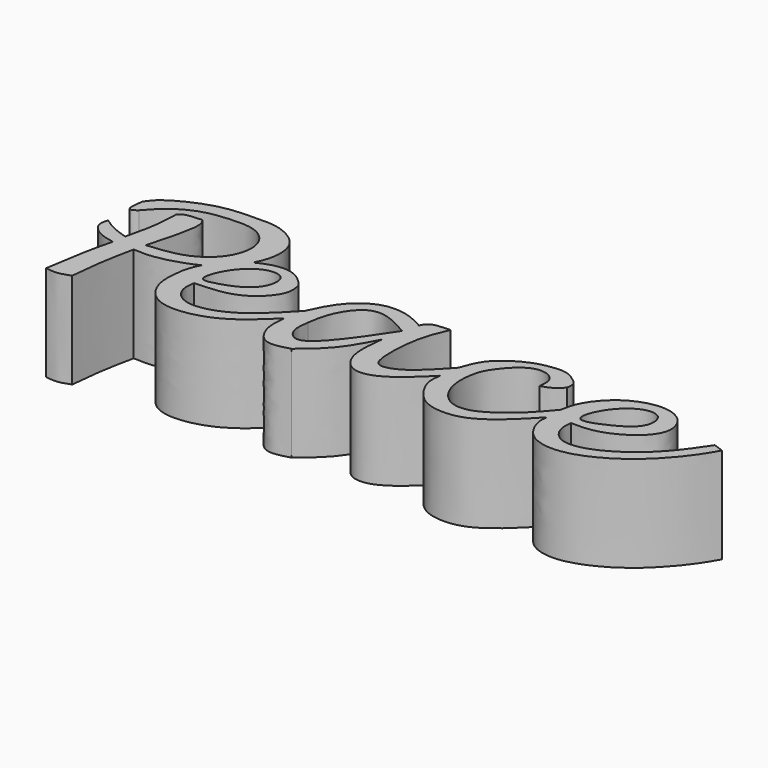
from build123d import *

# Parameters (mm, degrees)
F1_DEPTH = 15


with BuildPart() as f1:
    # F0 (on Top) → F1 (new body)
    with BuildSketch(Plane.XY):
        with BuildLine():
            add(Edge.make_bspline(
                [(-29.5197498053, 16.0896964371), (-29.2959248841, 17.0866768453), (-28.9570431175, 17.9865364975), (-28.5339232006, 18.7932092998)],
                knots=[0, 0, 0, 0, 0.1193114698, 0.1193114698, 0.1193114698, 0.1193114698], degree=3))
            add(Edge.make_bspline(
                [(-29.5197498053, 16.0896964371), (-29.7031065197, 14.6563172426), (-30.080045439, 11.7096217462), (-28.1322871252, 8.759925381), (-26.4865215868, 8.0765383318)],
                knots=[0, 0, 0, 0, 0.2073575456, 0.4262790671, 0.4262790671, 0.4262790671, 0.4262790671], degree=3))
            add(Edge.make_bspline(
                [(-26.4865215868, 8.0765383318), (-24.3712413413, 7.1981901762), (-17.8840994319, 8.2079095342), (-13.895871726, 12.139582434), (-11.8636386469, 14.1429975629)],
                knots=[0.4262790671, 0.4262790671, 0.4262790671, 0.4262790671, 0.7076559455, 1, 1, 1, 1], degree=3))
            add(Edge.make_bspline(
                [(-11.8636386469, 14.1429975629), (-11.9919670944, 13.0883304188), (-12.2526083771, 10.9462504463), (-10.2153785321, 7.2023382975), (-7.5198727613, 7.9751970563), (-6.1371922493, 8.3716409281)],
                knots=[0, 0, 0, 0, 0.3208255575, 0.6516122221, 1, 1, 1, 1], degree=3))
            add(Edge.make_bspline(
                [(-6.1371922493, 8.3716409281), (-4.7049770612, 9.5508191577), (-1.8004106416, 11.944123887), (0.0085061179, 15.4262155687), (0.9252529708, 17.1948950738)],
                knots=[0, 0, 0, 0, 0.4928718937, 1, 1, 1, 1], degree=3))
            add(Edge.make_bspline(
                [(0.9252529708, 17.1948950738), (0.7002885074, 15.2129187205), (0.2948956357, 11.6686773245), (2.8534995196, 8.3256503296), (7.2214848398, 9.0430540833), (10.5903189017, 12.2451424426), (12.4796722084, 14.1429975629)],
                knots=[0, 0, 0, 0, 0.2662560325, 0.4748550688, 0.6918347611, 1, 1, 1, 1], degree=3))
            add(Edge.make_bspline(
                [(12.4796722084, 14.1429975629), (12.3567270292, 13.3382773369), (12.14040693, 11.6866274324), (14.1680771363, 8.3563764669), (16.6960843798, 6.843858018), (20.9356335968, 6.7199377707), (25.0508891214, 9.0723771082), (28.001238583, 12.0543664551), (29.5260921121, 13.7017956004)],
                knots=[0, 0, 0, 0, 0.1309459503, 0.2919621729, 0.4354540719, 0.6027228467, 0.784505056, 1, 1, 1, 1], degree=3))
            add(Edge.make_bspline(
                [(29.5260921121, 13.7017956004), (29.4494344459, 13.1510419203), (29.3115775332, 11.9578711835), (31.001212058, 8.2394328011), (36.1145843581, 7.0708416903), (42.2117822652, 9.6169760573), (46.573863691, 13.1346350854), (49.9266045093, 17.0857546913), (51.1581874034, 19.2222665215), (51.7203956842, 20.1976578683)],
                knots=[0, 0, 0, 0, 0.0899502167, 0.2212376244, 0.3723173697, 0.5483148575, 0.7139379788, 0.8700324828, 1, 1, 1, 1], degree=3))
            Line((51.7203956842, 20.1976578683), (50.1595586538, 20.7686945796))
            add(Edge.make_bspline(
                [(32.7983126044, 14.3592404202), (32.7153503568, 13.7323555449), (32.5362242327, 12.3788307643), (34.177987249, 9.747083146), (38.8427355373, 9.7604999377), (45.8804799663, 14.4091846262), (48.7479970496, 18.6708504577), (50.1595586538, 20.7686945796)],
                knots=[0, 0, 0, 0, 0.130090907, 0.2808829393, 0.4700062965, 0.7391057348, 1, 1, 1, 1], degree=3))
            add(Edge.make_bspline(
                [(29.588283971, 16.3035858423), (29.7616917917, 17.2053776187), (30.1627716399, 19.291157298), (33.5068853144, 23.2810073199), (38.1596043126, 24.8599408195), (41.2541002931, 24.2873570254), (43.0490114044, 22.683768941), (43.7218716906, 20.0178969278), (41.6710895913, 16.88834866), (36.7785570041, 14.2784160551), (34.0517720177, 14.3337871939), (32.7983126044, 14.3592404202)],
                knots=[0, 0, 0, 0, 0.1000330229, 0.231369205, 0.3598860143, 0.4603773571, 0.5477091259, 0.6387126974, 0.7479317597, 0.8841282645, 1, 1, 1, 1], degree=3))
            add(Edge.make_bspline(
                [(23.645831272, 19.6124818176), (23.7203833838, 20.2123241708), (23.8704148875, 21.3933142156), (22.6701217375, 22.8924812944), (19.5221839217, 23.1427632594), (16.3109184961, 19.4772592399), (15.2895614031, 17.2986171252), (14.8792866219, 13.0982142101), (17.05717861, 9.3483199148), (21.2088747712, 8.5887501402), (26.7442270709, 12.8463793621), (28.7028105399, 15.2281055095), (29.588283971, 16.3035858423)],
                knots=[0, 0, 0, 0, 0.0707743039, 0.1396140029, 0.228929762, 0.3440556474, 0.4292761333, 0.536753367, 0.6438866817, 0.7459339665, 0.8852224949, 1, 1, 1, 1], degree=3))
            add(Edge.make_bspline(
                [(26.526927948, 21.3411394507), (26.1385483593, 20.9400395262), (25.3505362754, 20.126218212), (24.2194502874, 19.7853498294), (23.645831272, 19.6124818176)],
                knots=[0, 0, 0, 0, 0.4928599404, 1, 1, 1, 1], degree=3))
            add(Edge.make_bspline(
                [(12.8943044692, 17.1948950738), (13.3425896626, 18.491787842), (14.2804655004, 21.2142228005), (18.8593458781, 23.903692294), (21.393850445, 24.4249510687), (24.0737893185, 24.6930231444), (25.7581339132, 23.4584551751), (26.7110830768, 22.704102983), (26.5899543358, 21.8076092017), (26.526927948, 21.3411394507)],
                knots=[0, 0, 0, 0, 0.1840283222, 0.3856193225, 0.5329945244, 0.6763715981, 0.8040129767, 0.8980060108, 1, 1, 1, 1], degree=3))
            add(Edge.make_bspline(
                [(5.9051825665, 24.39795807), (5.2796526411, 22.9712299099), (3.9353644531, 19.9050894014), (3.7075616843, 12.9009672388), (4.9490431647, 11.3184163953), (8.496299722, 12.3856851943), (11.2468870531, 15.3909715866), (12.8943044692, 17.1948950738)],
                knots=[0, 0, 0, 0, 0.2170119072, 0.4664184993, 0.5823552154, 0.7497429619, 1, 1, 1, 1], degree=3))
            add(Edge.make_bspline(
                [(2.1475991234, 22.9039788246), (2.3428401586, 23.3003573055), (2.8310561944, 24.2915338294), (4.7522735677, 24.358045116), (5.9051825665, 24.39795807)],
                knots=[0, 0, 0, 0, 0.3999070512, 1, 1, 1, 1], degree=3))
            add(Edge.make_bspline(
                [(-11.1623937264, 17.1948950738), (-10.5398511892, 18.5628349484), (-9.2707374001, 21.3594980591), (-5.248213519, 24.7374533554), (-0.7298831893, 24.4906309653), (1.2322453903, 23.4086829672), (2.1475991234, 22.9039788246)],
                knots=[0, 0, 0, 0, 0.2603156398, 0.5312425545, 0.7812722516, 1, 1, 1, 1], degree=3))
            add(Edge.make_bspline(
                [(-26.3120550662, 14.4988177344), (-26.4222931202, 13.7768911895), (-26.6615542892, 12.2101495597), (-24.3282508745, 9.2469865739), (-17.4297661724, 10.5963680293), (-13.3925098593, 14.8444387075), (-11.1623937264, 17.1948950738)],
                knots=[0, 0, 0, 0, 0.1694155161, 0.367717612, 0.6506295652, 1, 1, 1, 1], degree=3))
            add(Edge.make_bspline(
                [(-15.95112037, 21.9937769871), (-15.7966520892, 21.216655299), (-15.4154688091, 19.2989425314), (-19.5008131736, 14.743263195), (-23.9492657643, 14.5836147697), (-26.3120550662, 14.4988177344)],
                knots=[0, 0, 0, 0, 0.2421048194, 0.5974450468, 1, 1, 1, 1], degree=3))
            add(Edge.make_bspline(
                [(-24.0700956622, 23.2628666258), (-23.2776920759, 23.6864516212), (-20.1311153039, 24.8738854789), (-17.7451969535, 24.2725213112), (-15.95112037, 21.9937769871)],
                knots=[0.4293270672, 0.4293270672, 0.4293270672, 0.4293270672, 0.5741513965, 1, 1, 1, 1], degree=3))
            add(Edge.make_bspline(
                [(-28.5339232006, 18.7932092998), (-27.4805344869, 19.3586454328), (-25.8445145474, 20.5733086864), (-24.5247192992, 22.4099469585), (-24.0700956622, 23.2628666258)],
                knots=[0.2164607486, 0.2164607486, 0.2164607486, 0.2164607486, 0.2921979477, 0.349944774, 0.349944774, 0.349944774, 0.349944774], degree=3))
        make_face()
        with BuildLine():
            add(Edge.make_bspline(
                [(-26.1831432581, 16.0770304501), (-26.5705475824, 16.5915824541), (-25.5236781222, 19.8500439887), (-22.3942558617, 22.7980811841), (-19.5909944076, 22.9806135847), (-18.455931748, 21.7897345319), (-18.7610605958, 19.3004890899), (-20.8794412927, 17.1979951748), (-24.0654910281, 16.0934411171), (-25.8961329296, 15.6958221609), (-26.1831432581, 16.0770304501)],
                knots=[0, 0, 0, 0, 0.1402941833, 0.3022737646, 0.4209424648, 0.5087922195, 0.6222593339, 0.7517086902, 0.8960623898, 1, 1, 1, 1], degree=3))
        make_face(mode=Mode.SUBTRACT)
        with BuildLine():
            add(Edge.make_bspline(
                [(-8.9235752821, 15.0464298204), (-9.0646859983, 14.0808295866), (-9.3271993781, 12.2844884749), (-7.5404688212, 10.3547407663), (-5.0207003169, 11.4635558948), (-1.2953094882, 16.3396092098), (0.5618805634, 19.1479797333), (1.4483764535, 20.4885043204)],
                knots=[0, 0, 0, 0, 0.1779548177, 0.3310557971, 0.4918670148, 0.7574519621, 1, 1, 1, 1], degree=3))
            add(Edge.make_bspline(
                [(-8.9235752821, 15.0464298204), (-8.7718449134, 16.1215699221), (-8.449567237, 18.4051843159), (-5.958882275, 22.3564152791), (-2.6113827935, 22.7845317726), (-0.0046509708, 21.3102749358), (1.4483764535, 20.4885043204)],
                knots=[0, 0, 0, 0, 0.2372477596, 0.5039179524, 0.7234771856, 1, 1, 1, 1], degree=3))
        make_face(mode=Mode.SUBTRACT)
        with BuildLine():
            add(Edge.make_bspline(
                [(32.9581163824, 15.9508809447), (32.4202349789, 16.4558861758), (33.5372547907, 19.9580854994), (37.2715590249, 23.1501136882), (40.5087156051, 22.7034723084), (40.7973008496, 19.1294802461), (37.0761086127, 16.8016116704), (33.520287852, 15.4230702953), (32.9581163824, 15.9508809447)],
                knots=[0, 0, 0, 0, 0.1648006178, 0.3622570844, 0.4996763079, 0.6407463677, 0.8277571879, 1, 1, 1, 1], degree=3))
        make_face(mode=Mode.SUBTRACT)
        with BuildLine():
            add(Edge.make_bspline(
                [(-37.63435781, 16.8396867812), (-36.792774095, 16.780997693), (-34.7988064496, 16.6419460296), (-30.9505530887, 17.6314034567), (-28.9442923194, 18.5729320891), (-28.5339232006, 18.7932092998)],
                knots=[0, 0, 0, 0, 0.0785934067, 0.1869557735, 0.2164607486, 0.2164607486, 0.2164607486, 0.2164607486], degree=3))
            add(Edge.make_bspline(
                [(-28.5339232006, 18.7932092998), (-27.4345002025, 20.8892454247), (-25.7663401568, 22.3561270188), (-24.0700956622, 23.2628666258)],
                knots=[0.1193114698, 0.1193114698, 0.1193114698, 0.1193114698, 0.4293270672, 0.4293270672, 0.4293270672, 0.4293270672], degree=3))
            add(Edge.make_bspline(
                [(-24.0700956622, 23.2628666258), (-23.6593076141, 24.0335463196), (-22.7421148215, 26.4102337749), (-23.137984421, 30.4038791076), (-27.4676487416, 32.7905284602), (-31.2729050018, 32.6073591163), (-36.826013927, 32.6764343172), (-43.5764893816, 29.296188472), (-44.3511297111, 27.8653610127), (-44.7214916348, 27.40371041)],
                knots=[0.349944774, 0.349944774, 0.349944774, 0.349944774, 0.4021235525, 0.501487602, 0.6002895059, 0.6916758101, 0.8050336314, 0.932529676, 1, 1, 1, 1], degree=3))
            add(Edge.make_bspline(
                [(-44.7214916348, 27.40371041), (-44.8994629954, 26.0626483288), (-45.0946801171, 24.4835341745), (-44.1135664101, 24.9118394746), (-43.5886271298, 25.354931131)],
                knots=[0, 0, 0, 0, 0.5888424904, 1, 1, 1, 1], degree=3))
            add(Edge.make_bspline(
                [(-43.5886271298, 25.354931131), (-42.8698733446, 26.1771232695), (-41.3516522159, 27.9138368734), (-37.6044812798, 30.0075770022), (-33.4805276823, 30.4938502102), (-29.1108568661, 30.5796693033), (-26.2024184332, 27.6396314104), (-26.8391241832, 22.8646700552), (-31.1110959696, 19.1945600689), (-35.1137430617, 18.8342796295), (-37.1904708445, 18.6473522335)],
                knots=[0, 0, 0, 0, 0.1099985997, 0.2323496608, 0.3556770614, 0.4783969704, 0.5912201693, 0.7150692357, 0.8521669233, 1, 1, 1, 1], degree=3))
            add(Edge.make_bspline(
                [(-37.1904708445, 18.6473522335), (-36.2452841246, 22.0915778581), (-34.9373760502, 26.85754675), (-35.7489373077, 27.8983428661), (-35.9740070999, 28.1869862229)],
                knots=[0, 0, 0, 0, 0.7226706054, 1, 1, 1, 1], degree=3))
            add(Edge.make_bspline(
                [(-35.9740070999, 28.1869862229), (-36.9473854974, 28.1461458568), (-38.5225068768, 28.0800579573), (-39.1300566376, 27.578966837), (-39.3621586263, 27.3875351995)],
                knots=[0, 0, 0, 0, 0.6179704055, 1, 1, 1, 1], degree=3))
            add(Edge.make_bspline(
                [(-40.5884683132, 18.8792515546), (-40.2150467083, 20.4148384075), (-39.4958540428, 23.3723073574), (-39.4055666832, 26.0838761589), (-39.3621586263, 27.3875351995)],
                knots=[0, 0, 0, 0, 0.519223322, 1, 1, 1, 1], degree=3))
            add(Edge.make_bspline(
                [(-44.8954962194, 20.8873717549), (-44.2531018535, 20.4531410381), (-42.9511384226, 19.5730702534), (-41.3829206703, 19.1125494232), (-40.5884683132, 18.8792515546)],
                knots=[0, 0, 0, 0, 0.4934043082, 1, 1, 1, 1], degree=3))
            add(Edge.make_bspline(
                [(-40.9114956856, 16.8396867812), (-41.8524511704, 17.0332486566), (-43.6302677156, 17.3989593732), (-45.3793010236, 19.2701406063), (-45.0464709781, 20.3827031771), (-44.8954962194, 20.8873717549)],
                knots=[0, 0, 0, 0, 0.3805574121, 0.7190151655, 1, 1, 1, 1], degree=3))
            add(Edge.make_bspline(
                [(-42.9034940898, 6.2811863609), (-42.5282867495, 8.7092642449), (-41.8715441541, 12.9592401912), (-41.1995633303, 15.6753381611), (-40.9114956856, 16.8396867812)],
                knots=[0, 0, 0, 0, 0.5713156768, 1, 1, 1, 1], degree=3))
            add(Edge.make_bspline(
                [(-39.1709432006, 6.7238314077), (-39.8278750159, 6.4831096726), (-41.0996635916, 6.0170839064), (-42.3156266432, 6.1951155046), (-42.9034940898, 6.2811863609)],
                knots=[0, 0, 0, 0, 0.5165416862, 1, 1, 1, 1], degree=3))
            add(Edge.make_bspline(
                [(-39.1709432006, 6.7238314077), (-39.0103435648, 8.4121673837), (-38.6882375031, 11.7983721501), (-37.986309728, 15.1560976908), (-37.63435781, 16.8396867812)],
                knots=[0, 0, 0, 0, 0.4985924043, 1, 1, 1, 1], degree=3))
        make_face()
        with BuildLine():
            add(Edge.make_bspline(
                [(-28.5339232006, 18.7932092998), (-27.4345002025, 20.8892454247), (-25.7663401568, 22.3561270188), (-24.0700956622, 23.2628666258)],
                knots=[0.1193114698, 0.1193114698, 0.1193114698, 0.1193114698, 0.4293270672, 0.4293270672, 0.4293270672, 0.4293270672], degree=3))
            add(Edge.make_bspline(
                [(-28.5339232006, 18.7932092998), (-27.4805344869, 19.3586454328), (-25.8445145474, 20.5733086864), (-24.5247192992, 22.4099469585), (-24.0700956622, 23.2628666258)],
                knots=[0.2164607486, 0.2164607486, 0.2164607486, 0.2164607486, 0.2921979477, 0.349944774, 0.349944774, 0.349944774, 0.349944774], degree=3))
        make_face()
    extrude(amount=F1_DEPTH)


solid = f1.part
